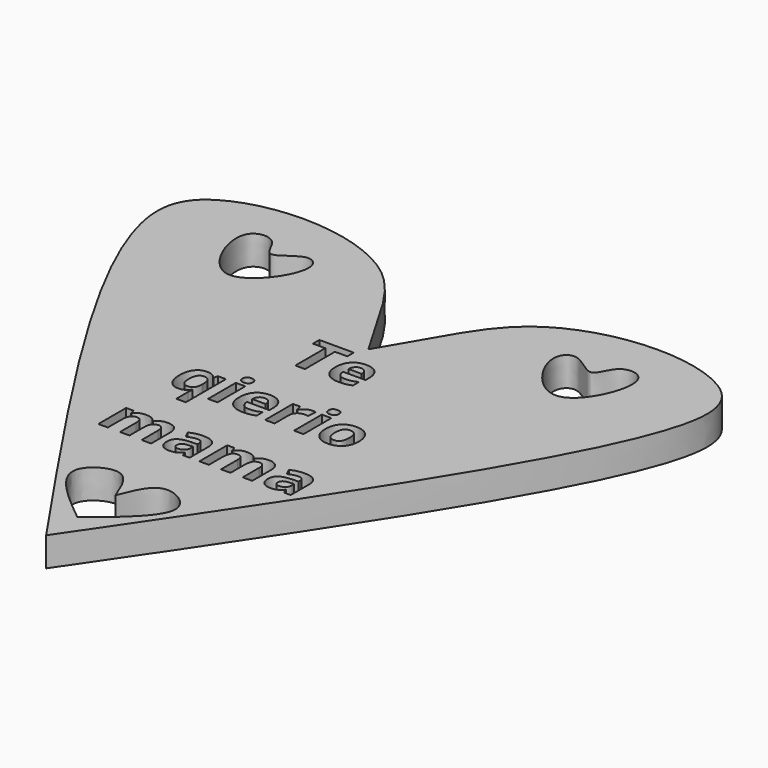
from build123d import *

# Parameters (mm, degrees)
F1_DEPTH     = 4
F2_TEXT_SIZE = 8.750537213
F3_DEPTH     = 25


# Not quite as in the source:
# - Text() gives the source's letters only with a copy of the font that has no kerning and outlines rounded to 1/6400 em; it was checked with that copy


with BuildPart() as f1:
    # F0 (on Top) → F1 (new body)
    with BuildSketch(Plane.XY):
        with BuildLine():
            add(Edge.make_bspline(
                [(0, 1.5368066961), (1.3336573158, 3.8458892136), (4.13759149, 8.7005961198), (9.4887028715, 17.6626513918), (21.8443199409, 21.737838825), (33.6686499139, 20.0030387889), (43.6345880228, 10.1467279068), (18.7664477324, -26.2909641997), (0, -53.7882372737)],
                knots=[0, 0, 0, 0, 0.1170093196, 0.2460050465, 0.3900423589, 0.5282261303, 0.6439814331, 1, 1, 1, 1], degree=3))
            add(Edge.make_bspline(
                [(0, 1.5368066961), (-1.3336573158, 3.8458892136), (-4.13759149, 8.7005961198), (-9.4887028715, 17.6626513918), (-21.8443199409, 21.737838825), (-33.6686499139, 20.0030387889), (-43.6345880228, 10.1467279068), (-18.7664477324, -26.2909641997), (0, -53.7882372737)],
                knots=[0, 0, 0, 0, 0.1170093196, 0.2460050465, 0.3900423589, 0.5282261303, 0.6439814331, 1, 1, 1, 1], degree=3))
        make_face()
        with BuildLine():
            add(Edge.make_bspline(
                [(0, -41.8779850006), (-0.8008003475, -39.81205216), (-2.3367241354, -35.8496220685), (-9.9245569101, -40.347691606), (-3.7508475, -45.3625984734), (0, -48.4094135463)],
                knots=[0, 0, 0, 0, 0.2994796015, 0.5743976577, 1, 1, 1, 1], degree=3))
            add(Edge.make_bspline(
                [(0, -41.8779850006), (0.8008003475, -39.81205216), (2.3367241354, -35.8496220685), (9.9245569101, -40.347691606), (3.7508475, -45.3625984734), (0, -48.4094135463)],
                knots=[0, 0, 0, 0, 0.2994796015, 0.5743976577, 1, 1, 1, 1], degree=3))
        make_face(mode=Mode.SUBTRACT)
        with BuildLine():
            add(Edge.make_bspline(
                [(-21.9955462962, 12.2944535688), (-22.7399405495, 12.4387097207), (-23.233503716, 15.7002330308), (-29.2424760108, 15.0237662415), (-23.2953585718, 0.8416280644), (-15.2336013116, 12.0184909315), (-18.5616374409, 15.1544722673), (-21.1709741144, 12.1346597372), (-21.9955462962, 12.2944535688)],
                knots=[0, 0, 0, 0, 0.1352489621, 0.2708734598, 0.5029731562, 0.7276893228, 0.8501835133, 1, 1, 1, 1], degree=3))
        make_face(mode=Mode.SUBTRACT)
        with BuildLine():
            add(Edge.make_bspline(
                [(21.9955462962, 12.2944535688), (22.7399405495, 12.4387097207), (23.233503716, 15.7002330308), (29.2424760108, 15.0237662415), (23.2953585718, 0.8416280644), (15.2336013116, 12.0184909315), (18.5616374409, 15.1544722673), (21.1709741144, 12.1346597372), (21.9955462962, 12.2944535688)],
                knots=[0, 0, 0, 0, 0.1352489621, 0.2708734598, 0.5029731562, 0.7276893228, 0.8501835133, 1, 1, 1, 1], degree=3))
        make_face(mode=Mode.SUBTRACT)
    extrude(amount=F1_DEPTH)

    # F2 (on face) → F3 (cut)
    with BuildSketch(Plane.XY.offset(4)):
        with Locations((-5.6367062542, -6.3003867933)):
            Text('Te', F2_TEXT_SIZE, font='Open Sans', font_style=FontStyle.BOLD, text_align=(TextAlign.LEFT, TextAlign.BOTTOM))
        with Locations((-12.458023466, -18.201117403)):
            Text('qierio', F2_TEXT_SIZE, font='Open Sans', font_style=FontStyle.BOLD, text_align=(TextAlign.LEFT, TextAlign.BOTTOM))
        with Locations((-12.458023466, -30.1018480126)):
            Text('mama', F2_TEXT_SIZE, font='Open Sans', font_style=FontStyle.BOLD, text_align=(TextAlign.LEFT, TextAlign.BOTTOM))
    extrude(amount=-F3_DEPTH, mode=Mode.SUBTRACT)


solid = f1.part
